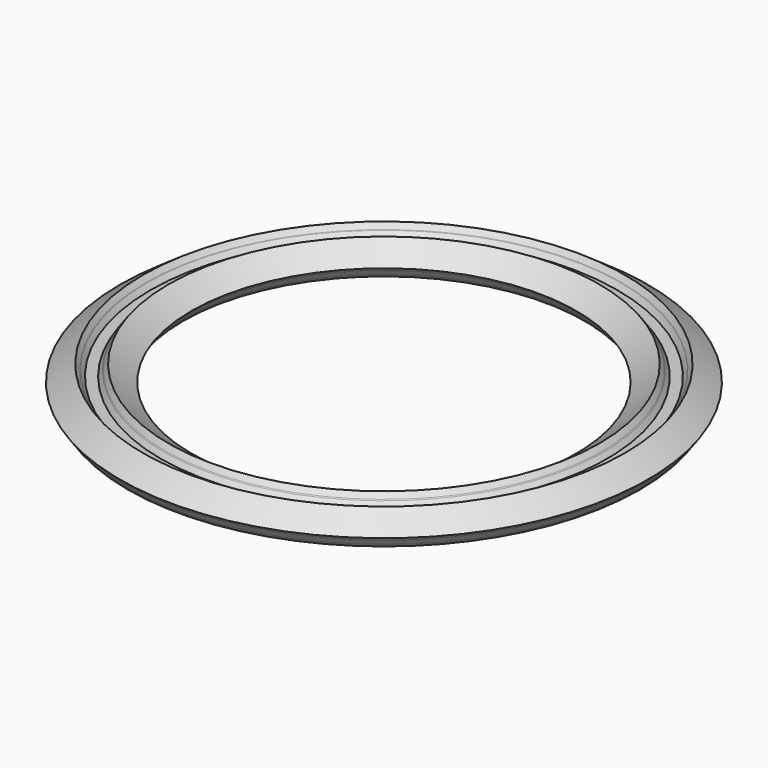
from build123d import *

# Parameters (mm, degrees)
F2_DEPTH      = 5
F2_DEPTH_BACK = 5
F4_DEPTH      = 5
F4_DEPTH_BACK = 5


with BuildPart() as f1:
    # F0 (on Front) → F1 (revolve)
    with BuildSketch(Plane.XZ):
        Polygon((-113.5293307371, 4.9221746135), (-112.67156485, 3.6916309601), (-108.5697526721, 6.5508505839), (-104.4679404942, 9.4100702078), (-103.7606077985, 8.3953367326), (-102.1198829273, 9.5390245822), (-103.6849815102, 11.7843017107), align=None)
        Polygon((-112.67156485, 3.6916309601), (-110.9560330757, 1.2305436534), (-106.8542208978, 4.0897632772), (-108.5697526721, 6.5508505839), align=None)
        Polygon((-87.8229461793, 6.5629257279), (-83.744250038, 3.6708265272), (-82.8766202778, 4.8944353695), (-92.6654910168, 11.8354734514), (-94.2561455773, 9.5921905737), (-92.6246671208, 8.4353508934), (-91.9016423206, 9.4550249287), align=None)
        Polygon((-110.9560330757, 1.2305436534), (-110.0982671885, 0), (-86.3471393187, 0), (-85.4795095585, 1.2236088424), (-89.5582056997, 4.1157080432), (-93.636901841, 7.0078072439), (-92.9138770408, 8.0274812792), (-94.5453554973, 9.1843209595), (-96.0139631617, 7.113159496), (-100.4289032436, 7.113159496), (-101.8153462856, 9.1021389036), (-103.4560711568, 7.958451054), (-102.7524087199, 6.9489829011), (-106.8542208978, 4.0897632772), align=None)
        Polygon((-101.9694497359, 9.323214404), (-102.1198829273, 9.5390245822), (-103.7606077985, 8.3953367326), (-103.6101746071, 8.1795265544), align=None)
        Polygon((-103.6101746071, 8.1795265544), (-103.4560711568, 7.958451054), (-101.8153462856, 9.1021389036), (-101.9694497359, 9.323214404), align=None)
        Polygon((-94.5453554973, 9.1843209595), (-92.9138770408, 8.0274812792), (-92.7692720808, 8.2314160863), (-94.4007505373, 9.3882557666), align=None)
        Polygon((-92.6246671208, 8.4353508934), (-94.2561455773, 9.5921905737), (-94.4007505373, 9.3882557666), (-92.7692720808, 8.2314160863), align=None)
        Polygon((-89.5582056997, 4.1157080432), (-85.4795095585, 1.2236088424), (-83.744250038, 3.6708265272), (-87.8229461793, 6.5629257279), align=None)
        Polygon((-108.5697526721, 6.5508505839), (-106.8542208978, 4.0897632772), (-102.7524087199, 6.9489829011), (-103.4560711568, 7.958451054), (-103.6101746071, 8.1795265544), (-103.7606077985, 8.3953367326), (-104.4679404942, 9.4100702078), align=None)
        Polygon((-93.636901841, 7.0078072439), (-89.5582056997, 4.1157080432), (-87.8229461793, 6.5629257279), (-91.9016423206, 9.4550249287), (-92.6246671208, 8.4353508934), (-92.7692720808, 8.2314160863), (-92.9138770408, 8.0274812792), align=None)
    revolve(axis=Axis((0, 0, 10.2496305481), (0, 0, 1)))

    # F0 (on Front) → F2 (cut, two sides)
    with BuildSketch(Plane.XZ) as f2_sk:
        Polygon((-112.67156485, 3.6916309601), (-110.9560330757, 1.2305436534), (-106.8542208978, 4.0897632772), (-108.5697526721, 6.5508505839), align=None)
    extrude(amount=F2_DEPTH, mode=Mode.SUBTRACT)
    extrude(f2_sk.sketch, amount=-F2_DEPTH_BACK, mode=Mode.SUBTRACT)

    # F0 (on Front) → F3 (revolve, cut)
    with BuildSketch(Plane.XZ):
        Polygon((-108.5697526721, 6.5508505839), (-106.8542208978, 4.0897632772), (-102.7524087199, 6.9489829011), (-103.4560711568, 7.958451054), (-103.6101746071, 8.1795265544), (-103.7606077985, 8.3953367326), (-104.4679404942, 9.4100702078), align=None)
    revolve(axis=Axis((-107.7119867849, 0, 5.3203069306), (0.5718439248, 0, -0.8203624356)), mode=Mode.SUBTRACT)


with BuildPart() as f4:
    # F0 (on Front) → F4 (new body, two sides)
    with BuildSketch(Plane.XZ) as f4_sk:
        Polygon((-89.5582056997, 4.1157080432), (-85.4795095585, 1.2236088424), (-83.744250038, 3.6708265272), (-87.8229461793, 6.5629257279), align=None)
    extrude(amount=F4_DEPTH)
    extrude(f4_sk.sketch, amount=-F4_DEPTH_BACK)

    # F0 (on Front) → F5 (revolve)
    with BuildSketch(Plane.XZ):
        Polygon((-93.636901841, 7.0078072439), (-89.5582056997, 4.1157080432), (-87.8229461793, 6.5629257279), (-91.9016423206, 9.4550249287), (-92.6246671208, 8.4353508934), (-92.7692720808, 8.2314160863), (-92.9138770408, 8.0274812792), align=None)
    revolve(axis=Axis((-88.6905759395, 0, 5.3393168855), (-0.5784198402, 0, -0.8157392283)))


solid = Compound([f1.part, f4.part])
